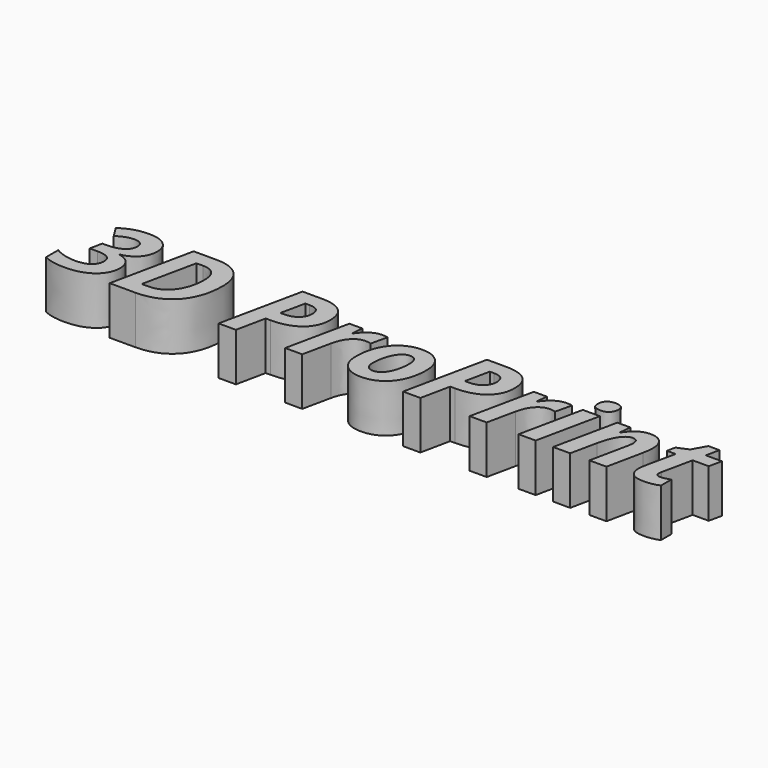
from build123d import *

# Parameters (mm, degrees)
F0_TEXT_SIZE = 61.4592702025
F1_DEPTH     = 25.4


# Not quite as in the source:
# - Text() gives the source's letters only with a copy of the font that has no kerning and outlines rounded to 1/6400 em; it was checked with that copy


with BuildPart() as f1:
    # F0 (on Top) → F1 (new body)
    with BuildSketch(Plane.XY):
        with Locations((-68.8875317574, -10.165695101)):
            Text('3D ProPrint', F0_TEXT_SIZE, font='Open Sans', font_style=FontStyle.BOLDITALIC, text_align=(TextAlign.LEFT, TextAlign.BOTTOM))
    extrude(amount=F1_DEPTH)


solid = f1.part
